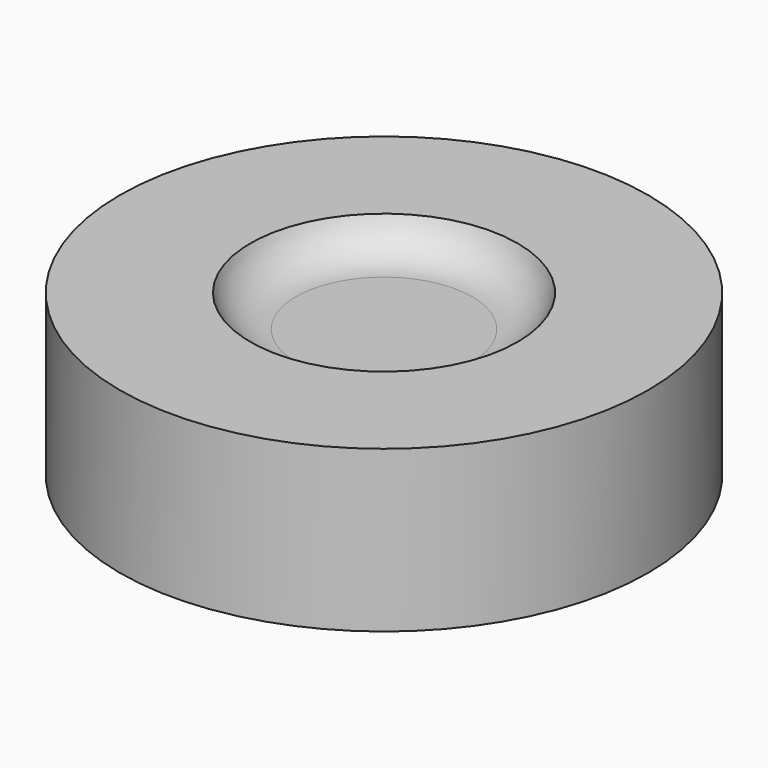
from build123d import *

# Parameters (mm, degrees)
F0_R     = 41.7000635609
F1_DEPTH = 25.4
F2_R     = 21.0958969827
F3_DEPTH = 5.08


# Not quite as in the source:
# - a fillet or chamfer that OpenCascade refuses, or shapes differently, is made with other operations: its cross-section is extruded or revolved along the edge and cut away or added


with BuildPart() as f1:
    # F0 (on Top) → F1 (new body)
    with BuildSketch(Plane.XY):
        Circle(F0_R)
    extrude(amount=-F1_DEPTH)

    # F2 (on face) → F3 (cut)
    with BuildSketch(Plane.XY):
        Circle(F2_R)
    extrude(amount=-F3_DEPTH, mode=Mode.SUBTRACT)

    # F4: fillet of radius 7.62 on 1 edges, made by hand

    # F4_s1 → F4_t2 (revolve)
    with BuildSketch(Plane.XZ):
        with BuildLine():
            ThreePointArc((21.0958969827, 0), (18.3111011371, -3.6817039467), (13.9116920859, -5.08))
            Line((13.9116920859, -5.08), (21.0958969827, -5.08))
            Line((21.0958969827, -5.08), (21.0958969827, 0))
        make_face()
    revolve(axis=Axis((0, 0, -5.08), (0, 0, 1)))


solid = f1.part
